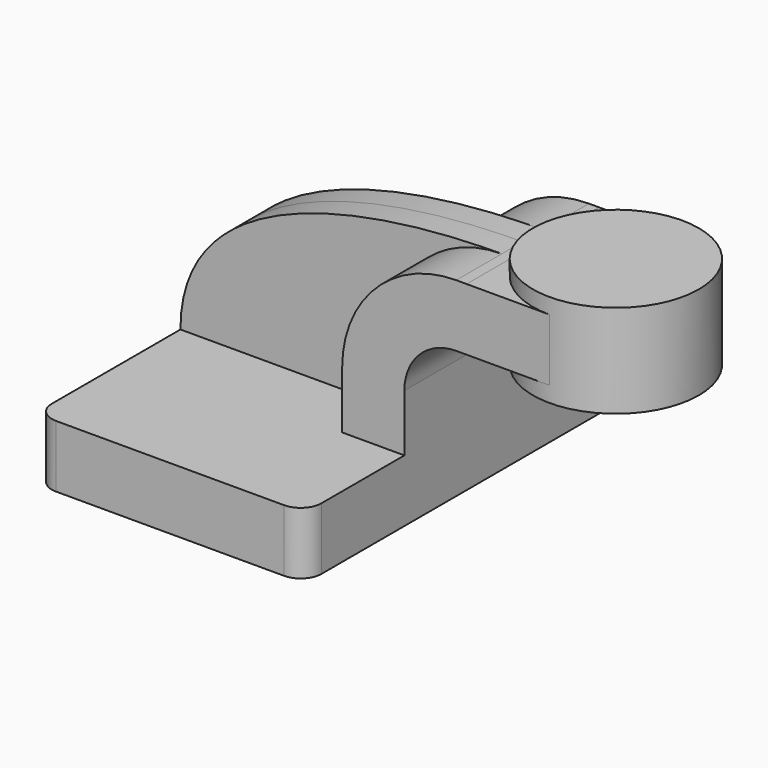
from build123d import *

# Parameters (mm, degrees)
F1_DEPTH = 63.5
F0_W     = 25.3999010601
F0_H     = 19.05
F2_DEPTH = 25.4
F3_DEPTH = 7.9375
F5_R     = 6.35


# Not quite as in the source:
# - ends of sketch curves that miss each other by under 0.0002 mm in the source are joined


with BuildPart() as f1:
    # F0 (on Front) → F1 (new body, symmetric)
    with BuildSketch(Plane.XZ):
        Polygon((22.225, 9.525), (-41.275, 9.525), (-41.275, -9.525), (41.275, -9.525), (41.275, 9.525), align=None)
    extrude(amount=F1_DEPTH, both=True)

    # F0 (on Front) → F2 (join, symmetric)
    with BuildSketch(Plane.XZ):
        with Locations((73.0249505301, 52.4002)):
            Rectangle(F0_W, F0_H)
        with BuildLine():
            Line((22.225, 27.0002), (22.225, 9.5249091869))
            Line((22.225, 9.5249091869), (41.275, 9.525))
            Line((41.275, 9.525), (41.275, 27.0002))
            ThreePointArc((41.275, 27.0002), (45.9246798487, 38.2255201513), (57.15, 42.8752))
            Line((57.15, 42.8752), (60.325, 42.8752))
            Line((60.325, 42.8752), (60.325, 61.9252))
            add(Edge.make_bspline(
                [(57.15, 61.9252), (59.3391618347, 61.9252), (59.4645664096, 61.9133971632), (60.325, 61.9252)],
                knots=[0.8556201459, 0.8556201459, 0.8556201459, 0.8556201459, 1, 1, 1, 1], degree=3))
            ThreePointArc((57.15, 61.9252), (32.4542956671, 51.6959043329), (22.225, 27.0002))
        make_face()
    extrude(amount=F2_DEPTH, both=True)

    # F0 (on Front) → F3 (join, symmetric)
    with BuildSketch(Plane.XZ):
        with BuildLine():
            add(Edge.make_bspline(
                [(-41.275, 9.525), (-41.2749116122, 61.5106898116), (44.1766459292, 61.9252), (57.15, 61.9252)],
                knots=[0, 0, 0, 0, 0.8556201459, 0.8556201459, 0.8556201459, 0.8556201459], degree=3))
            Line((-41.275, 9.525), (22.225, 9.525))
            Line((22.225, 9.525), (22.225, 27.0002))
            ThreePointArc((22.225, 27.0002), (32.4542956671, 51.6959043329), (57.15, 61.9252))
        make_face()
    extrude(amount=F3_DEPTH, both=True)

    # F0 (on Front) → F4 (revolve)
    with BuildSketch(Plane.XZ):
        Polygon((85.725, 66.675), (85.725, 61.9252), (85.725, 42.8752), (85.725, 38.1), (111.125, 38.1), (111.125, 66.675), align=None)
    revolve(axis=Axis((85.725, 0, 52.3875), (0, 0, 1)))

    # F5
    f5_edges = [f1.edges().sort_by_distance(p)[0] for p in [
        (41.275, -63.5, 0),
        (-41.275, -63.5, 0),
        (41.275, 63.5, 0),
        (-41.275, 63.5, 0),
    ]]
    fillet(f5_edges, radius=F5_R)


solid = f1.part
